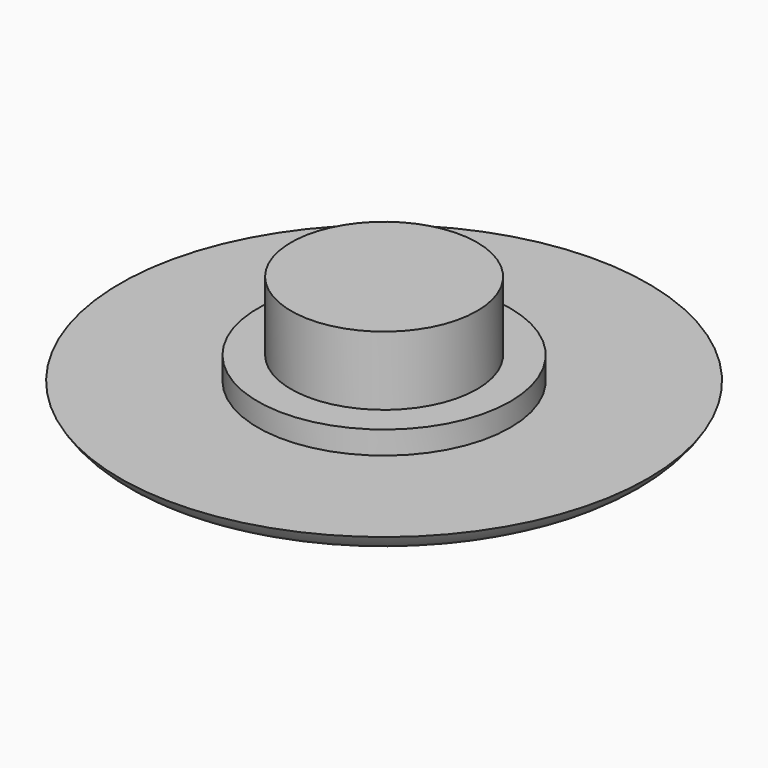
from build123d import *

# Parameters (mm, degrees)
F0_R     = 11.5
F0_R_2   = 5.5
F1_DEPTH = 1
F0_R_3   = 4.05
F2_DEPTH = 2
F0_R_4   = 2
F3_DEPTH = 5


# Not quite as in the source:
# - a fillet or chamfer that OpenCascade refuses, or shapes differently, is made with other operations: its cross-section is extruded or revolved along the edge and cut away or added


with BuildPart() as f1:
    # F0 (on Top) → F1 (new body)
    with BuildSketch(Plane.XY):
        Circle(F0_R)
        Circle(F0_R_2, mode=Mode.SUBTRACT)
    extrude(amount=F1_DEPTH)

    # F0 (on Top) → F2 (join)
    with BuildSketch(Plane.XY):
        Circle(F0_R_2)
        Circle(F0_R_3, mode=Mode.SUBTRACT)
    extrude(amount=F2_DEPTH)

    # F0 (on Top) → F3 (join)
    with BuildSketch(Plane.XY):
        Circle(F0_R_3)
        Circle(F0_R_4, mode=Mode.SUBTRACT)
        Circle(F0_R_4)
    extrude(amount=F3_DEPTH)

    # F4: fillet of radius 2 on 1 edges, made by hand

    # F4_s1 → F4_t2 (revolve, cut)
    with BuildSketch(Plane.XZ):
        with BuildLine():
            ThreePointArc((11.5, 1), (10.7679491924, 0.2679491924), (9.7679491924, 0))
            Line((9.7679491924, 0), (11.5, 0))
            Line((11.5, 0), (11.5, 1))
        make_face()
    revolve(axis=Axis((0, 0, 0), (0, 0, 1)), mode=Mode.SUBTRACT)


solid = f1.part
